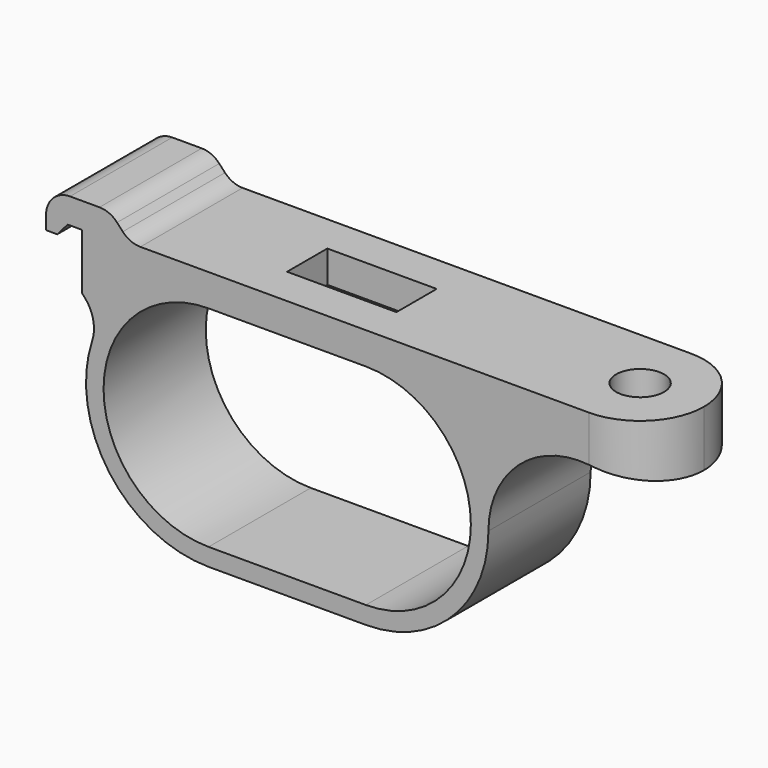
from build123d import *

# Parameters (mm, degrees)
F1_DEPTH = 16
F2_R     = 3
F3_R     = 7.99999
F4_R     = 3
F4_W     = 13.7
F4_H     = 6.3
F5_DEPTH = 10


# Not quite as in the source:
# - a fillet or chamfer is up to 0.001 mm smaller than in the source, because OpenCascade refuses the exact size


with BuildPart() as f1:
    # F0 (on Front) → F1 (new body)
    with BuildSketch(Plane.XZ):
        with BuildLine():
            ThreePointArc((-25.7, 9.65), (-24.3502481093, 7.4100162997), (-24.4315048785, 4.7960624973))
            ThreePointArc((-24.4315048785, 4.7960624973), (-22.2846704688, -9.0000816848), (-9.85, -15.35))
            Line((-9.85, -15.35), (9.85, -15.35))
            ThreePointArc((9.85, -15.35), (20.7040890912, -10.8540890912), (25.2, 0))
            ThreePointArc((25.2, 0), (29.210075991, 8.7034493587), (38.4314464174, 11.3105680079))
            Line((38.4314464174, 11.3105680079), (45.8, 10.15))
            Line((45.8, 10.15), (45.8, 17.15))
            Line((45.8, 17.15), (-19.7, 17.15))
            Line((-19.7, 17.15), (-22.2, 19.85))
            Line((-22.2, 19.85), (-30.2, 19.85))
            Line((-30.2, 19.85), (-30.2, 15.15))
            Line((-30.2, 15.15), (-28.8, 15.15))
            Line((-28.8, 15.15), (-27.5, 16.65))
            Line((-27.5, 16.65), (-25.7, 16.65))
            Line((-25.7, 16.65), (-25.7, 9.65))
        make_face()
        with BuildLine():
            ThreePointArc((-9.85, -13.15), (-23, 0), (-9.85, 13.15))
            Line((-9.85, 13.15), (9.85, 13.15))
            ThreePointArc((9.85, 13.15), (23, 0), (9.85, -13.15))
            Line((9.85, -13.15), (-9.85, -13.15))
        make_face(mode=Mode.SUBTRACT)
    extrude(amount=F1_DEPTH)

    # F2
    f2_edges = [f1.edges().sort_by_distance(p)[0] for p in [
        (-30.2, -8, 19.85),
        (-22.2, -8, 19.85),
        (-19.7, -8, 17.15),
    ]]
    fillet(f2_edges, radius=F2_R)

    # F3 (radius 8 in the source; OpenCascade refuses exactly that, so slightly less here)
    f3_edges = [f1.edges().sort_by_distance(p)[0] for p in [
        (45.8, -16, 13.65),
        (45.8, 0, 13.65),
    ]]
    fillet(f3_edges, radius=F3_R)

    # F4 (on face) → F5 (cut)
    with BuildSketch(Plane.XY.offset(17.15)):
        with Locations((37.8, -8)):
            Circle(F4_R)
        with Locations((2.95, -8)):
            Rectangle(F4_W, F4_H)
    extrude(amount=-F5_DEPTH, mode=Mode.SUBTRACT)


solid = f1.part
